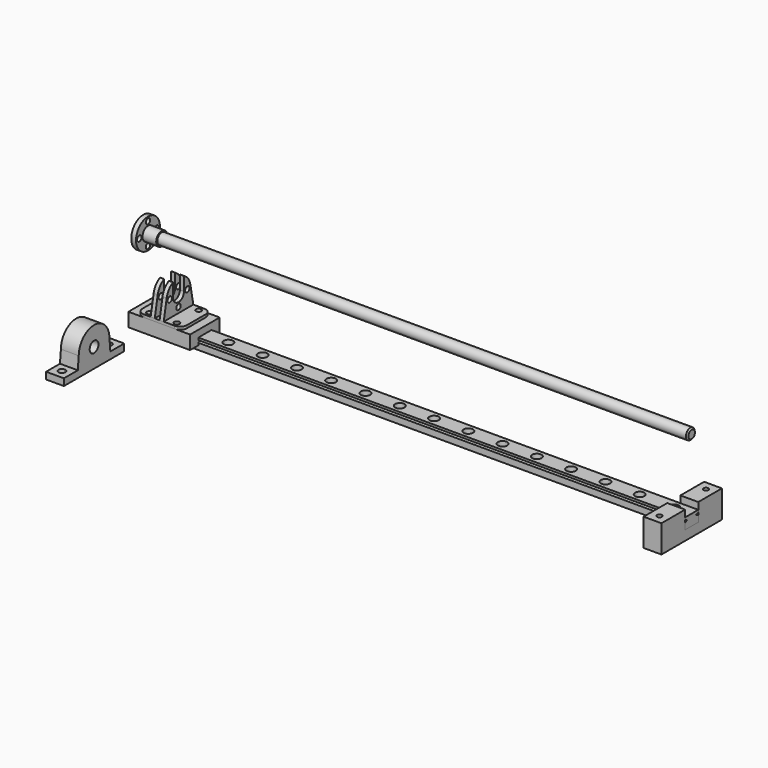
from build123d import *

# Parameters (mm, degrees)
F1_DEPTH         = 400
F2_R             = 3.425
F2_R_2           = 2.1
F3_DEPTH         = 5
F4_DEPTH         = 8
F5_DEPTH         = 45
F7_D             = 4
F7_DEPTH         = 5
F7_TIP           = 1.2017212381
F6_R             = 2
F6_W             = 3
F6_H             = 27
F6_W_2           = 3.5
F8_DEPTH         = 2
F9_DEPTH         = 26
F10_R            = 2
F11_DEPTH        = 9.5
F12_DEPTH        = 1.5
F13_DEPTH        = 13.5
F0_R             = 2
F14_DEPTH        = 3.5
F15_DEPTH        = 400
F0_R_2           = 5.9
F0_R_3           = 4
F16_DEPTH        = 13
F19_D            = 5
F19_DEPTH        = 5
F19_TIP          = 1.5021515476
F19_ON_F17_D     = 5
F19_ON_F17_DEPTH = 5
F19_ON_F17_TIP   = 1.5021515476
F21_SIZE         = 1
F23_DEPTH        = 13
F25_D            = 3.6
F25_CBORE_D      = 9
F25_CBORE_DEPTH  = 4
F26_D            = 3.6
F26_CBORE_D      = 9
F26_CBORE_DEPTH  = 17


# Not quite as in the source:
# - a feature names something its author has since deleted; it is built from what else it names


with BuildPart() as f1:
    # F0 (on Right) → F1 (new body)
    with BuildSketch(Plane.YZ):
        Polygon((0, 3), (0, 0), (6, 0), (6, 8), (0, 8), (0, 6.3572470099), (1.9986690022, 5.520161707), (0, 4.683076404), align=None)
        Polygon((6, 8), (6, 0), (12, 0), (12, 3), (12, 4.683076404), (10.0013309978, 5.520161707), (12, 6.3572470099), (12, 8), align=None)
    extrude(amount=F1_DEPTH)

    # F2 (on face) → F3 (cut)
    with BuildSketch(Plane.XY.offset(8)):
        with Locations((12.125, 6)):
            Circle(F2_R)
        with Locations((12.125, 6)):
            Circle(F2_R_2, mode=Mode.SUBTRACT)
        with Locations((37.125, 6)):
            Circle(F2_R)
        with Locations((37.125, 6)):
            Circle(F2_R_2, mode=Mode.SUBTRACT)
        with Locations((62.125, 6)):
            Circle(F2_R)
        with Locations((62.125, 6)):
            Circle(F2_R_2, mode=Mode.SUBTRACT)
        with Locations((87.125, 6)):
            Circle(F2_R)
        with Locations((87.125, 6)):
            Circle(F2_R_2, mode=Mode.SUBTRACT)
        with BuildLine():
            ThreePointArc((115.55, 6), (112.125, 9.425), (108.7, 6))
            ThreePointArc((108.7, 6), (112.125, 2.575), (115.55, 6))
        make_face()
        with BuildLine():
            ThreePointArc((114.225, 6), (112.125, 3.9), (110.025, 6))
            ThreePointArc((110.025, 6), (112.125, 8.1), (114.225, 6))
        make_face(mode=Mode.SUBTRACT)
        with Locations((137.125, 6)):
            Circle(F2_R)
        with Locations((137.125, 6)):
            Circle(F2_R_2, mode=Mode.SUBTRACT)
        with Locations((162.125, 6)):
            Circle(F2_R)
        with Locations((162.125, 6)):
            Circle(F2_R_2, mode=Mode.SUBTRACT)
        with Locations((187.125, 6)):
            Circle(F2_R)
        with Locations((187.125, 6)):
            Circle(F2_R_2, mode=Mode.SUBTRACT)
        with Locations((387.125, 6)):
            Circle(F2_R)
        with Locations((387.125, 6)):
            Circle(F2_R_2, mode=Mode.SUBTRACT)
        with Locations((362.125, 6)):
            Circle(F2_R)
        with Locations((362.125, 6)):
            Circle(F2_R_2, mode=Mode.SUBTRACT)
        with Locations((337.125, 6)):
            Circle(F2_R)
        with Locations((337.125, 6)):
            Circle(F2_R_2, mode=Mode.SUBTRACT)
        with Locations((312.125, 6)):
            Circle(F2_R)
        with Locations((312.125, 6)):
            Circle(F2_R_2, mode=Mode.SUBTRACT)
        with Locations((287.125, 6)):
            Circle(F2_R)
        with Locations((287.125, 6)):
            Circle(F2_R_2, mode=Mode.SUBTRACT)
        with Locations((262.125, 6)):
            Circle(F2_R)
        with Locations((262.125, 6)):
            Circle(F2_R_2, mode=Mode.SUBTRACT)
        with Locations((237.125, 6)):
            Circle(F2_R)
        with Locations((237.125, 6)):
            Circle(F2_R_2, mode=Mode.SUBTRACT)
        with Locations((212.125, 6)):
            Circle(F2_R)
        with Locations((212.125, 6)):
            Circle(F2_R_2, mode=Mode.SUBTRACT)
        with Locations((12.125, 6)):
            Circle(F2_R_2)
        with Locations((37.125, 6)):
            Circle(F2_R_2)
        with Locations((62.125, 6)):
            Circle(F2_R_2)
        with Locations((87.125, 6)):
            Circle(F2_R_2)
        with BuildLine():
            ThreePointArc((114.225, 6), (112.125, 8.1), (110.025, 6))
            ThreePointArc((110.025, 6), (112.125, 3.9), (114.225, 6))
        make_face()
        with Locations((137.125, 6)):
            Circle(F2_R_2)
        with Locations((162.125, 6)):
            Circle(F2_R_2)
        with Locations((187.125, 6)):
            Circle(F2_R_2)
        with Locations((387.125, 6)):
            Circle(F2_R_2)
        with Locations((362.125, 6)):
            Circle(F2_R_2)
        with Locations((337.125, 6)):
            Circle(F2_R_2)
        with Locations((312.125, 6)):
            Circle(F2_R_2)
        with Locations((287.125, 6)):
            Circle(F2_R_2)
        with Locations((262.125, 6)):
            Circle(F2_R_2)
        with Locations((237.125, 6)):
            Circle(F2_R_2)
        with Locations((212.125, 6)):
            Circle(F2_R_2)
    extrude(amount=-F3_DEPTH, mode=Mode.SUBTRACT)

    # F2 (on face) → F4 (cut, through all)
    with BuildSketch(Plane.XY.offset(8)):
        with Locations((12.125, 6)):
            Circle(F2_R_2)
        with Locations((37.125, 6)):
            Circle(F2_R_2)
        with Locations((62.125, 6)):
            Circle(F2_R_2)
        with Locations((87.125, 6)):
            Circle(F2_R_2)
        with BuildLine():
            ThreePointArc((114.225, 6), (112.125, 8.1), (110.025, 6))
            ThreePointArc((110.025, 6), (112.125, 3.9), (114.225, 6))
        make_face()
        with Locations((137.125, 6)):
            Circle(F2_R_2)
        with Locations((162.125, 6)):
            Circle(F2_R_2)
        with Locations((187.125, 6)):
            Circle(F2_R_2)
        with Locations((212.125, 6)):
            Circle(F2_R_2)
        with Locations((237.125, 6)):
            Circle(F2_R_2)
        with Locations((262.125, 6)):
            Circle(F2_R_2)
        with Locations((287.125, 6)):
            Circle(F2_R_2)
        with Locations((312.125, 6)):
            Circle(F2_R_2)
        with Locations((337.125, 6)):
            Circle(F2_R_2)
        with Locations((362.125, 6)):
            Circle(F2_R_2)
        with Locations((387.125, 6)):
            Circle(F2_R_2)
    extrude(amount=-F4_DEPTH, mode=Mode.SUBTRACT)


with BuildPart() as f5:
    # F0 (on Right) → F5 (new body)
    with BuildSketch(Plane.YZ):
        Polygon((-7.5, 3), (0, 3), (0, 4.683076404), (0, 6.3572470099), (0, 8), (6, 8), (6, 13), (-7.5, 13), align=None)
        Polygon((6, 13), (6, 8), (12, 8), (12, 6.3572470099), (12, 4.683076404), (12, 3), (19.5, 3), (19.5, 13), align=None)
        Polygon((0, 6.3572470099), (0, 4.683076404), (1.9986690022, 5.520161707), align=None)
        Polygon((10.0013309978, 5.520161707), (12, 4.683076404), (12, 6.3572470099), align=None)
    extrude(amount=F5_DEPTH)

    # F7
    with Locations(Plane.XY.offset(13)):
        with Locations((12.5, 16), (32.5, 16), (32.5, -4), (12.5, -4)):
            Hole(F7_D / 2, depth=F7_DEPTH)
            with Locations((0, 0, -(F7_DEPTH + F7_TIP / 2))):  # 118° drill point
                Cone(0, F7_D / 2, F7_TIP, mode=Mode.SUBTRACT)


with BuildPart() as f8:
    # F6 (on face) → F8 (new body)
    with BuildSketch(Plane.XY.offset(13)):
        with BuildLine():
            Line((12.5, 19.5), (11.25, 19.5))
            ThreePointArc((11.25, 19.5), (7.7144660941, 18.0355339059), (6.25, 14.5))
            Line((6.25, 14.5), (6.25, -2.5))
            ThreePointArc((6.25, -2.5), (7.7144660941, -6.0355339059), (11.25, -7.5))
            Line((11.25, -7.5), (16.25, -7.5))
            Line((16.25, -7.5), (16.25, 19.5))
            Line((16.25, 19.5), (12.5, 19.5))
        make_face()
        with Locations((12.5, -4)):
            Circle(F6_R, mode=Mode.SUBTRACT)
        with Locations((12.5, 16)):
            Circle(F6_R, mode=Mode.SUBTRACT)
        with Locations((17.75, 6)):
            Rectangle(F6_W, F6_H)
        with Locations((21, 6)):
            Rectangle(F6_W_2, F6_H)
        with Locations((24.25, 6)):
            Rectangle(F6_W, F6_H)
        with BuildLine():
            Line((33.75, 19.5), (25.75, 19.5))
            Line((25.75, 19.5), (25.75, -7.5))
            Line((25.75, -7.5), (33.75, -7.5))
            ThreePointArc((33.75, -7.5), (37.2855339059, -6.0355339059), (38.75, -2.5))
            Line((38.75, -2.5), (38.75, 14.5))
            ThreePointArc((38.75, 14.5), (38.6920886291, 15.2587884964), (38.5196960071, 16))
            ThreePointArc((38.5196960071, 16), (36.7080398915, 18.5311288741), (33.75, 19.5))
        make_face()
        with Locations((32.5, -4)):
            Circle(F6_R, mode=Mode.SUBTRACT)
        with Locations((32.5, 16)):
            Circle(F6_R, mode=Mode.SUBTRACT)
    extrude(amount=F8_DEPTH)

    # F6 (on face) → F9 (join)
    with BuildSketch(Plane.XY.offset(13)):
        with Locations((24.25, 6)):
            Rectangle(F6_W, F6_H)
        with Locations((17.75, 6)):
            Rectangle(F6_W, F6_H)
    extrude(amount=F9_DEPTH)

    # F10 (on face) → F11 (cut, through all)
    with BuildSketch(Plane.YZ.offset(25.75)):
        with BuildLine():
            ThreePointArc((1, 27), (6, 32), (11, 27))
            Line((11, 27), (11, 36.7979589711))
            ThreePointArc((11, 36.7979589711), (6, 38), (1, 36.7979589711))
            Line((1, 36.7979589711), (1, 27))
        make_face()
        with Locations((6, 35)):
            Circle(F10_R, mode=Mode.SUBTRACT)
        with BuildLine():
            ThreePointArc((1, 36.7979589711), (6, 38), (11, 36.7979589711))
            Line((11, 36.7979589711), (11, 39))
            Line((11, 39), (1, 39))
            Line((1, 39), (1, 36.7979589711))
        make_face()
        with BuildLine():
            ThreePointArc((1, 27), (6, 22), (11, 27))
            ThreePointArc((11, 27), (6, 32), (1, 27))
        make_face()
        with BuildLine():
            ThreePointArc((-4.8033852543, 29.0704750777), (-2.7957517134, 33.6056605874), (1, 36.7979589711))
            Line((1, 36.7979589711), (1, 39))
            Line((1, 39), (-7.5, 39))
            Line((-7.5, 39), (-7.5, 15))
            Line((-7.5, 15), (-4.8033852543, 29.0704750777))
        make_face()
        with BuildLine():
            Line((11, 39), (11, 36.7979589711))
            ThreePointArc((11, 36.7979589711), (14.7957517134, 33.6056605874), (16.8033852543, 29.0704750777))
            Line((16.8033852543, 29.0704750777), (19.5, 15))
            Line((19.5, 15), (19.5, 39))
            Line((19.5, 39), (11, 39))
        make_face()
        with Locations((6, 35)):
            Circle(F10_R)
        with Locations((14, 27)):
            Circle(F10_R)
        with Locations((6, 19)):
            Circle(F10_R)
        with Locations((-2, 27)):
            Circle(F10_R)
    extrude(amount=-F11_DEPTH, mode=Mode.SUBTRACT)


with BuildPart() as f12:
    # F0 (on Right) → F12 (new body)
    with BuildSketch(Plane.YZ):
        with BuildLine():
            ThreePointArc((11, 58.8707253337), (2.4644660941, 62.4062592396), (6, 53.8707253337))
            ThreePointArc((6, 53.8707253337), (9.5355339059, 55.3351914278), (11, 58.8707253337))
        make_face()
        with BuildLine():
            ThreePointArc((10, 58.8707253337), (8.8284271247, 56.0422982089), (6, 54.8707253337))
            ThreePointArc((6, 54.8707253337), (3.1715728753, 61.6991524584), (10, 58.8707253337))
        make_face(mode=Mode.SUBTRACT)
    extrude(amount=-F12_DEPTH)

    # F0 (on Right) → F13 (join)
    with BuildSketch(Plane.YZ):
        with BuildLine():
            ThreePointArc((11, 58.8707253337), (2.4644660941, 62.4062592396), (6, 53.8707253337))
            ThreePointArc((6, 53.8707253337), (9.5355339059, 55.3351914278), (11, 58.8707253337))
        make_face()
        with BuildLine():
            ThreePointArc((10, 58.8707253337), (8.8284271247, 56.0422982089), (6, 54.8707253337))
            ThreePointArc((6, 54.8707253337), (3.1715728753, 61.6991524584), (10, 58.8707253337))
        make_face(mode=Mode.SUBTRACT)
    extrude(amount=F13_DEPTH)

    # F0 (on Right) → F14 (join)
    with BuildSketch(Plane.YZ):
        with BuildLine():
            ThreePointArc((16.9, 58.8707253337), (-1.7074639149, 66.5781892486), (6, 47.9707253337))
            ThreePointArc((6, 47.9707253337), (13.7074639149, 51.1632614188), (16.9, 58.8707253337))
        make_face()
        with BuildLine():
            ThreePointArc((8, 50.9207253337), (7.4142135624, 49.5065117713), (6, 48.9207253337))
            ThreePointArc((6, 48.9207253337), (4, 50.9207253337), (6, 52.9207253337))
            ThreePointArc((6, 52.9207253337), (7.4142135624, 52.3349388961), (8, 50.9207253337))
        make_face(mode=Mode.SUBTRACT)
        with Locations((-1.95, 58.8707253337)):
            Circle(F0_R, mode=Mode.SUBTRACT)
        with BuildLine():
            ThreePointArc((11, 58.8707253337), (9.5355339059, 55.3351914278), (6, 53.8707253337))
            ThreePointArc((6, 53.8707253337), (2.4644660941, 62.4062592396), (11, 58.8707253337))
        make_face(mode=Mode.SUBTRACT)
        with Locations((13.95, 58.8707253337)):
            Circle(F0_R, mode=Mode.SUBTRACT)
        with Locations((6, 66.8207253337)):
            Circle(F0_R, mode=Mode.SUBTRACT)
    extrude(amount=F14_DEPTH)


with BuildPart() as f15:
    # F0 (on Right) → F15 (new body)
    with BuildSketch(Plane.YZ):
        with BuildLine():
            ThreePointArc((10, 58.8707253337), (3.1715728753, 61.6991524584), (6, 54.8707253337))
            ThreePointArc((6, 54.8707253337), (8.8284271247, 56.0422982089), (10, 58.8707253337))
        make_face()
    extrude(amount=F15_DEPTH)

    # F21
    f21_edges = [f15.edges().sort_by_distance(p)[0] for p in [
        (0, 6, 62.870725),
        (400, 6, 62.870725),
    ]]
    chamfer(f21_edges, length=F21_SIZE)


with BuildPart() as f16:
    # F0 (on Right) → F16 (new body)
    with BuildSketch(Plane.YZ):
        with BuildLine():
            Line((-55.0357139111, 0), (-27.5357139111, 0))
            Line((-27.5357139111, 0), (-27.5357139111, 5))
            Line((-27.5357139111, 5), (-40.1957139111, 5))
            Line((-40.1957139111, 5), (-41.0357139111, 14))
            ThreePointArc((-41.0357139111, 14), (-45.1362189744, 4.1005050634), (-55.0357139111, 0))
        make_face()
        with BuildLine():
            Line((-82.5357139111, 0), (-55.0357139111, 0))
            ThreePointArc((-55.0357139111, 0), (-64.9352088477, 4.1005050634), (-69.0357139111, 14))
            Line((-69.0357139111, 14), (-69.8757139111, 5))
            Line((-69.8757139111, 5), (-82.5357139111, 5))
            Line((-82.5357139111, 5), (-82.5357139111, 0))
        make_face()
        with BuildLine():
            ThreePointArc((-69.0357139111, 14), (-64.9352088477, 4.1005050634), (-55.0357139111, 0))
            ThreePointArc((-55.0357139111, 0), (-45.1362189744, 4.1005050634), (-41.0357139111, 14))
            ThreePointArc((-41.0357139111, 14), (-55.0357139111, 28), (-69.0357139111, 14))
        make_face()
        with Locations((-55.0357139111, 14)):
            Circle(F0_R_2, mode=Mode.SUBTRACT)
        with Locations((-55.0357139111, 14)):
            Circle(F0_R_2)
        with Locations((-55.0357139111, 14)):
            Circle(F0_R_3, mode=Mode.SUBTRACT)
    extrude(amount=F16_DEPTH)

    # F19
    with Locations(Plane.XY.offset(5)):
        with Locations((6.5, -76.2057139111)):
            Hole(F19_D / 2, depth=F19_DEPTH)
            with Locations((0, 0, -(F19_DEPTH + F19_TIP / 2))):  # 118° drill point
                Cone(0, F19_D / 2, F19_TIP, mode=Mode.SUBTRACT)

    # F19 on F17
    with Locations(Plane.XY.offset(5)):
        with Locations((6.5, -33.8657139111)):
            Hole(F19_ON_F17_D / 2, depth=F19_ON_F17_DEPTH)
            with Locations((0, 0, -(F19_ON_F17_DEPTH + F19_ON_F17_TIP / 2))):  # 118° drill point
                Cone(0, F19_ON_F17_D / 2, F19_ON_F17_TIP, mode=Mode.SUBTRACT)


with BuildPart() as f23:
    # F22 (on face) → F23 (new body)
    with BuildSketch(Plane.YZ.offset(400)):
        Polygon((6, -7.0792869665), (6, 0), (0, 0), (0, 4.683076404), (0, 6.3572470099), (0, 8), (0, 13), (-21.575, 13), (-21.575, -7.0792869665), align=None)
        Polygon((12, 0), (6, 0), (6, -7.0792869665), (33.575, -7.0792869665), (33.575, 13), (12, 13), (12, 8), (12, 6.3572470099), (12, 4.683076404), align=None)
    extrude(amount=-F23_DEPTH)

    # F25 (through all)
    with Locations(Plane(origin=(0, 0, -7.0792869665), x_dir=(1, 0, 0), z_dir=(0, 0, -1))):
        with Locations((393.5, -6)):
            CounterBoreHole(F25_D / 2, F25_CBORE_D / 2, F25_CBORE_DEPTH)

    # F26 (through all)
    with Locations(Plane(origin=(0, 0, -7.0792869665), x_dir=(1, 0, 0), z_dir=(0, 0, -1))):
        with Locations((393.5, 15.17), (393.5, -27.17)):
            CounterBoreHole(F26_D / 2, F26_CBORE_D / 2, F26_CBORE_DEPTH)


solid = Compound([f1.part, f5.part, f8.part, f12.part, f15.part, f16.part, f23.part])
